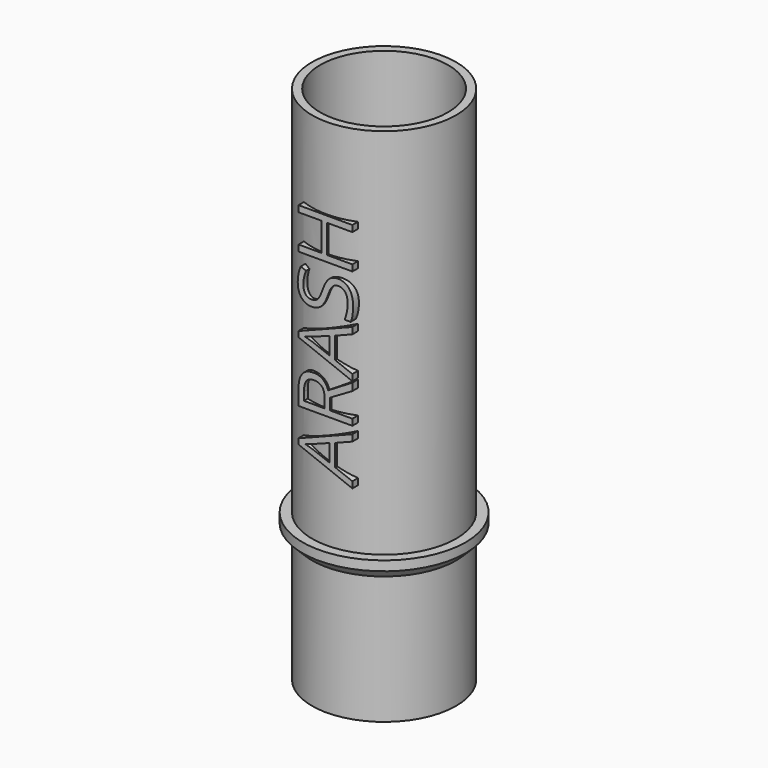
from build123d import *

# Parameters (mm, degrees)
F5_TEXT_SIZE = 23.5844828445
F6_DEPTH     = 3


# Not quite as in the source:
# - Text() gives the source's letters only with a copy of the font that has no kerning and outlines rounded to 1/6400 em; it was checked with that copy


with BuildPart() as f1:
    # F0 (on Front) → F1 (revolve)
    with BuildSketch(Plane.XZ):
        Polygon((20, 0), (0, 0), (0, -2.5), (22.5, -2.5), (22.5, 160), (20, 160), align=None)
    revolve(axis=Axis((0, 0, -1.25), (0, 0, 1)))

    # F2 (on Front) → F3 (revolve)
    with BuildSketch(Plane.XZ):
        Polygon((25.5, 43.5), (22.5, 43.5), (22.5, 37.5), (25.5, 40.5), align=None)
    revolve(axis=Axis((0, 0, 19.6070168167), (0, 0, 1)))

    # F5 (on offset) → F6 (join)
    with BuildSketch(Plane.XZ.offset(20)):
        with Locations(Location((8.490413824, 62.1205100976), (0, 0, 90))):
            Text('ARASH', F5_TEXT_SIZE, font='Open Sans', text_align=(TextAlign.LEFT, TextAlign.BOTTOM))
    extrude(amount=F6_DEPTH)


solid = f1.part
